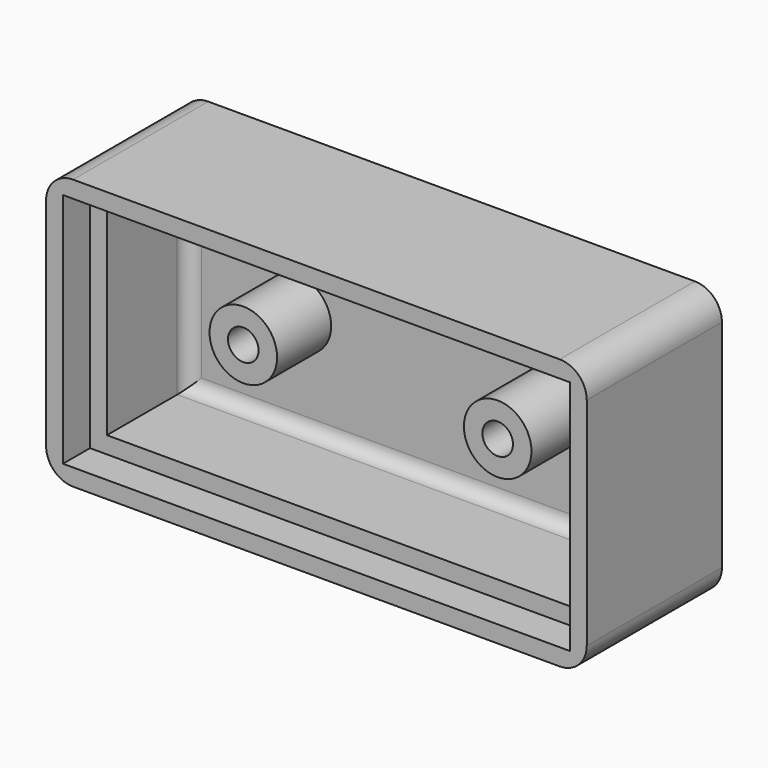
from build123d import *

# Parameters (mm, degrees)
F0_W     = 50.8
F0_H     = 25.4
F0_W_2   = 44.45
F0_H_2   = 19.05
F1_DEPTH = 12.7
F2_W     = 44.45
F2_H     = 19.05
F3_DEPTH = 9.525
F4_R     = 1.27
F5_W     = 50.8
F5_H     = 25.4
F5_W_2   = 47.625
F5_H_2   = 22.225
F6_DEPTH = 3.175
F7_R     = 2.54
F8_R     = 3.175
F8_R_2   = 1.43697608
F9_DEPTH = 6.35


with BuildPart() as f1:
    # F0 (on Front) → F1 (new body)
    with BuildSketch(Plane.XZ):
        Rectangle(F0_W, F0_H)
        Rectangle(F0_W_2, F0_H_2, mode=Mode.SUBTRACT)
        Rectangle(F0_W_2, F0_H_2)
    extrude(amount=F1_DEPTH)

    # F2 (on face) → F3 (cut)
    with BuildSketch(Plane.XZ.offset(12.7)):
        Rectangle(F2_W, F2_H)
    extrude(amount=-F3_DEPTH, mode=Mode.SUBTRACT)

    # F4
    f4_edges = [f1.edges().sort_by_distance(p)[0] for p in [
        (22.225, -3.175, 0),
        (0, -3.175, 9.525),
        (-22.225, -3.175, 0),
        (0, -3.175, -9.525),
    ]]
    fillet(f4_edges, radius=F4_R)

    # F5 (on face) → F6 (join)
    with BuildSketch(Plane.XZ.offset(12.7)):
        Rectangle(F5_W, F5_H)
        Rectangle(F5_W_2, F5_H_2, mode=Mode.SUBTRACT)
    extrude(amount=F6_DEPTH)

    # F7
    f7_edges = [f1.edges().sort_by_distance(p)[0] for p in [
        (25.4, -7.9375, 12.7),
        (25.4, -7.9375, -12.7),
        (-25.4, -7.9375, -12.7),
        (-25.4, -7.9375, 12.7),
    ]]
    fillet(f7_edges, radius=F7_R)

    # F8 (on face) → F9 (join)
    with BuildSketch(Plane.XZ.offset(3.175)):
        with Locations((11.9508895849, 0)):
            Circle(F8_R)
        with Locations((11.9508895849, 0)):
            Circle(F8_R_2, mode=Mode.SUBTRACT)
        with Locations((-11.9508895849, 0)):
            Circle(F8_R)
        with Locations((-11.9508895849, 0)):
            Circle(F8_R_2, mode=Mode.SUBTRACT)
    extrude(amount=F9_DEPTH)


solid = f1.part
